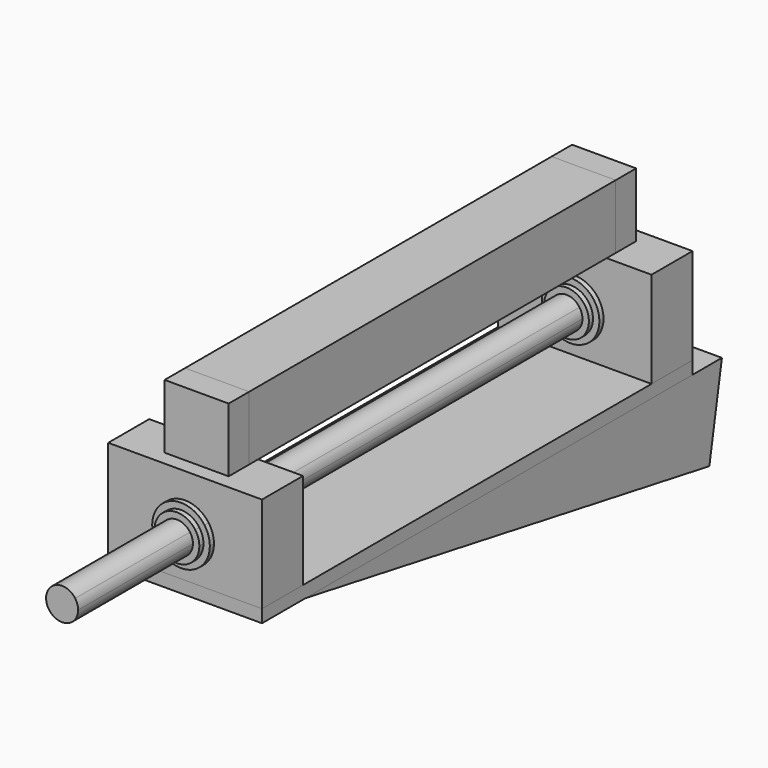
from build123d import *

# Parameters (mm, degrees)
F0_W          = 152.4
F0_H          = 533.4
F1_DEPTH      = 12.7
F2_W          = 152.4
F2_H          = 50.8
F3_DEPTH      = 95.25
F4_W          = 63.5
F4_H          = 25.4
F5_DEPTH      = 63.5
F7_DEPTH      = 482.6
F7_DEPTH_BACK = 152.4
F8_R          = 22.225
F9_DEPTH      = 10.16
F8_R_2        = 28.575
F10_DEPTH     = 5.08
F11_DEPTH     = 10.16
F12_DEPTH     = 5.08
F13_R         = 22.225
F14_DEPTH     = 10.16
F13_R_2       = 28.575
F15_DEPTH     = 5.08
F16_DEPTH     = 454.025
F18_DEPTH     = 152.4


with BuildPart() as f1:
    # F0 (on Top) → F1 (new body)
    with BuildSketch(Plane.XY):
        with Locations((76.2, -266.7)):
            Rectangle(F0_W, F0_H)
    extrude(amount=F1_DEPTH)


with BuildPart() as f3:
    # F2 (on face) → F3 (new body)
    with BuildSketch(Plane.XY.offset(12.7)):
        with Locations((76.2, -25.4)):
            Rectangle(F2_W, F2_H)
    extrude(amount=F3_DEPTH)


with BuildPart() as f3b:
    # F2 (on face) → F3, piece 2 (new body)
    with BuildSketch(Plane.XY.offset(12.7)):
        with Locations((76.2, -508)):
            Rectangle(F2_W, F2_H)
    extrude(amount=F3_DEPTH)


with BuildPart() as f5:
    # F4 (on face) → F5 (new body)
    with BuildSketch(Plane.XY.offset(107.95)):
        with Locations((76.2, -506.4125)):
            Rectangle(F4_W, F4_H)
    extrude(amount=F5_DEPTH)


with BuildPart() as f5b:
    # F4 (on face) → F5, piece 2 (new body)
    with BuildSketch(Plane.XY.offset(107.95)):
        with Locations((76.2, -26.9875)):
            Rectangle(F4_W, F4_H)
    extrude(amount=F5_DEPTH)


with BuildPart() as f7:
    # F6 (on face) → F7 (new body, two sides)
    with BuildSketch(Plane.XZ.offset(533.4)) as f7_sk:
        with BuildLine():
            ThreePointArc((63.2456113625, 63.1510252849), (60.325, 53.975), (63.2456113625, 44.7989747151))
            Line((63.2456113625, 44.7989747151), (76.2, 53.975))
            Line((76.2, 53.975), (63.2456113625, 63.1510252849))
        make_face()
        with BuildLine():
            Line((76.2, 53.975), (63.2456113625, 44.7989747151))
            ThreePointArc((63.2456113625, 44.7989747151), (76.2, 38.1), (89.1543886375, 44.7989747151))
            Line((89.1543886375, 44.7989747151), (76.2, 53.975))
        make_face()
        with BuildLine():
            Line((63.2456113625, 63.1510252849), (76.2, 53.975))
            Line((76.2, 53.975), (89.1543886375, 63.1510252849))
            ThreePointArc((89.1543886375, 63.1510252849), (76.2, 69.85), (63.2456113625, 63.1510252849))
        make_face()
        with BuildLine():
            Line((89.1543886375, 63.1510252849), (76.2, 53.975))
            Line((76.2, 53.975), (89.1543886375, 44.7989747151))
            ThreePointArc((89.1543886375, 44.7989747151), (91.3272361094, 49.1601944286), (92.075, 53.975))
            ThreePointArc((92.075, 53.975), (91.3272361094, 58.7898055714), (89.1543886375, 63.1510252849))
        make_face()
    extrude(amount=-F7_DEPTH)
    extrude(f7_sk.sketch, amount=F7_DEPTH_BACK)


with BuildPart() as f9:
    # F8 (on face) → F9 (new body)
    with BuildSketch(Plane.XZ.offset(50.8)):
        with Locations((76.2, 53.975)):
            Circle(F8_R)
    extrude(amount=F9_DEPTH)


with BuildPart() as f10:
    # F8 (on face) → F10 (new body)
    with BuildSketch(Plane.XZ.offset(50.8)):
        with Locations((76.2, 53.975)):
            Circle(F8_R_2)
        with Locations((76.2, 53.975)):
            Circle(F8_R, mode=Mode.SUBTRACT)
    extrude(amount=F10_DEPTH)


with BuildPart() as f11:
    # F6 (on face) → F11 (new body)
    with BuildSketch(Plane.XZ.offset(533.4)):
        with BuildLine():
            Line((63.2456113625, 44.7989747151), (58.0638559075, 41.1285646012))
            ThreePointArc((58.0638559075, 41.1285646012), (76.2, 31.75), (94.3361440925, 41.1285646012))
            Line((94.3361440925, 41.1285646012), (89.1543886375, 44.7989747151))
            ThreePointArc((89.1543886375, 44.7989747151), (76.2, 38.1), (63.2456113625, 44.7989747151))
        make_face()
        with BuildLine():
            ThreePointArc((58.0638559075, 66.8214353988), (53.975, 53.975), (58.0638559075, 41.1285646012))
            Line((58.0638559075, 41.1285646012), (63.2456113625, 44.7989747151))
            ThreePointArc((63.2456113625, 44.7989747151), (60.325, 53.975), (63.2456113625, 63.1510252849))
            Line((63.2456113625, 63.1510252849), (58.0638559075, 66.8214353988))
        make_face()
        with BuildLine():
            ThreePointArc((94.3361440925, 66.8214353988), (76.2, 76.2), (58.0638559075, 66.8214353988))
            Line((58.0638559075, 66.8214353988), (63.2456113625, 63.1510252849))
            ThreePointArc((63.2456113625, 63.1510252849), (76.2, 69.85), (89.1543886375, 63.1510252849))
            Line((89.1543886375, 63.1510252849), (94.3361440925, 66.8214353988))
        make_face()
        with BuildLine():
            Line((89.1543886375, 44.7989747151), (94.3361440925, 41.1285646012))
            ThreePointArc((94.3361440925, 41.1285646012), (97.3781305532, 47.2342722001), (98.425, 53.975))
            ThreePointArc((98.425, 53.975), (97.3781305532, 60.7157277999), (94.3361440925, 66.8214353988))
            Line((94.3361440925, 66.8214353988), (89.1543886375, 63.1510252849))
            ThreePointArc((89.1543886375, 63.1510252849), (91.3272361094, 58.7898055714), (92.075, 53.975))
            ThreePointArc((92.075, 53.975), (91.3272361094, 49.1601944286), (89.1543886375, 44.7989747151))
        make_face()
    extrude(amount=F11_DEPTH)


with BuildPart() as f12:
    # F6 (on face) → F12 (new body)
    with BuildSketch(Plane.XZ.offset(533.4)):
        with BuildLine():
            ThreePointArc((99.5178995475, 70.4918455128), (76.2, 82.55), (52.8821004525, 70.4918455128))
            Line((52.8821004525, 70.4918455128), (58.0638559075, 66.8214353988))
            ThreePointArc((58.0638559075, 66.8214353988), (76.2, 76.2), (94.3361440925, 66.8214353988))
            Line((94.3361440925, 66.8214353988), (99.5178995475, 70.4918455128))
        make_face()
        with BuildLine():
            ThreePointArc((52.8821004525, 70.4918455128), (47.625, 53.975), (52.8821004525, 37.4581544872))
            Line((52.8821004525, 37.4581544872), (58.0638559075, 41.1285646012))
            ThreePointArc((58.0638559075, 41.1285646012), (53.975, 53.975), (58.0638559075, 66.8214353988))
            Line((58.0638559075, 66.8214353988), (52.8821004525, 70.4918455128))
        make_face()
        with BuildLine():
            Line((58.0638559075, 41.1285646012), (52.8821004525, 37.4581544872))
            ThreePointArc((52.8821004525, 37.4581544872), (76.2, 25.4), (99.5178995475, 37.4581544872))
            Line((99.5178995475, 37.4581544872), (94.3361440925, 41.1285646012))
            ThreePointArc((94.3361440925, 41.1285646012), (76.2, 31.75), (58.0638559075, 41.1285646012))
        make_face()
        with BuildLine():
            Line((94.3361440925, 41.1285646012), (99.5178995475, 37.4581544872))
            ThreePointArc((99.5178995475, 37.4581544872), (103.429024997, 45.3083499716), (104.775, 53.975))
            ThreePointArc((104.775, 53.975), (103.429024997, 62.6416500284), (99.5178995475, 70.4918455128))
            Line((99.5178995475, 70.4918455128), (94.3361440925, 66.8214353988))
            ThreePointArc((94.3361440925, 66.8214353988), (97.3781305532, 60.7157277999), (98.425, 53.975))
            ThreePointArc((98.425, 53.975), (97.3781305532, 47.2342722001), (94.3361440925, 41.1285646012))
        make_face()
    extrude(amount=F12_DEPTH)


with BuildPart() as f14:
    # F13 (on face) → F14 (new body)
    with BuildSketch(Plane(origin=(0, -482.6, 0), x_dir=(-1, 0, 0), z_dir=(0, 1, 0))):
        with Locations((-76.2, 53.975)):
            Circle(F13_R)
    extrude(amount=F14_DEPTH)


with BuildPart() as f15:
    # F13 (on face) → F15 (new body)
    with BuildSketch(Plane(origin=(0, -482.6, 0), x_dir=(-1, 0, 0), z_dir=(0, 1, 0))):
        with Locations((-76.2, 53.975)):
            Circle(F13_R_2)
        with Locations((-76.2, 53.975)):
            Circle(F13_R, mode=Mode.SUBTRACT)
    extrude(amount=F15_DEPTH)


with BuildPart() as f16:
    # F16 (new, through all): a face of the model
    f16_faces = [f5.part.faces().sort_by_distance(p)[0] for p in [
        (76.2, -493.7125, 139.7),
    ]]
    extrude(f16_faces, amount=F16_DEPTH)


with BuildPart() as f18:
    # F17 (on face) → F18 (new body)
    with BuildSketch(Plane.YZ.offset(152.4)):
        Polygon((0, 0), (-479.425, 0), (20.8573385302, -88.2132742548), (36.411718838, 0), align=None)
    extrude(amount=-F18_DEPTH)


solid = Compound([f1.part, f3.part, f3b.part, f5.part, f5b.part, f7.part, f9.part, f10.part, f11.part, f12.part, f14.part, f15.part, f16.part, f18.part])
